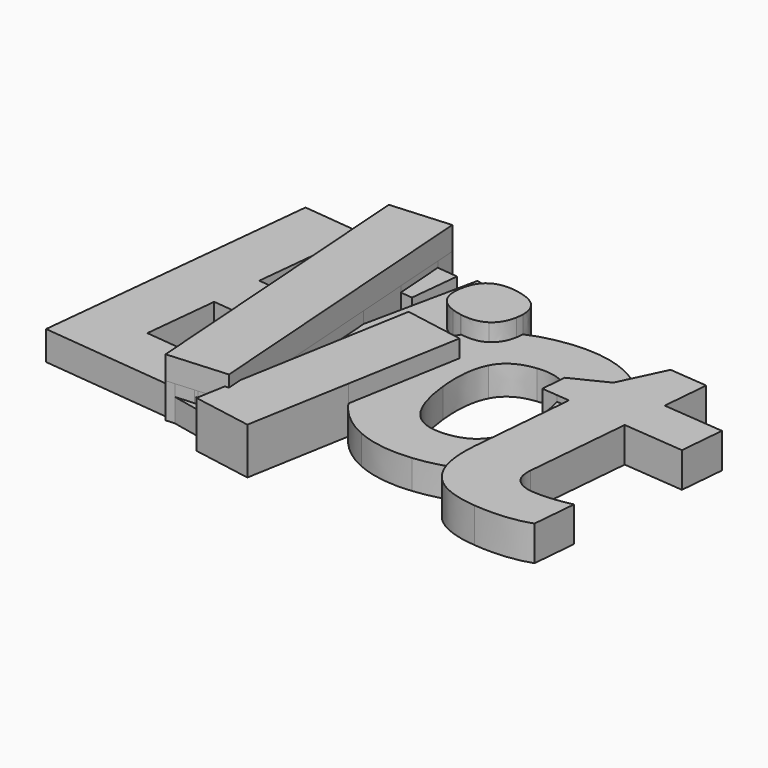
from build123d import *

# Parameters (mm, degrees)
F1_DEPTH = 2.5
F2_DEPTH = 3
F3_DEPTH = 2
F4_DEPTH = 4
F5_DEPTH = 2.5
F6_DEPTH = 3


# Not quite as in the source:
# - a feature names something its author has since deleted; it is built from what else it names


with BuildPart() as f1:
    # F0 (on Top) → F1 (new body)
    with BuildSketch(Plane.XY):
        Polygon((-35.3778718855, -10.0628526476), (-35.0793464958, -10.0938324205), (-35.073883926, -10.0411943399), align=None)
        Polygon((-36.9787601383, -10.1769115417), (-35.3778718855, -10.0628526476), (-37.0800270676, -9.8862097799), (-37.134769104, -10.1437508123), align=None)
        Polygon((-37.0800270676, -9.8862097799), (-35.3778718855, -10.0628526476), (-35.073883926, -10.0411943399), (-34.631335756, -5.7767387725), (-36.1725358308, -5.6167991831), align=None)
        Polygon((-37.7560246741, -9.8160574477), (-37.0800270676, -9.8862097799), (-36.1725358308, -5.6167991831), (-38.0692340227, -5.4199674186), align=None)
        Polygon((-49.2771882306, -8.6204371001), (-37.7560246741, -9.8160574477), (-38.0692340227, -5.4199674186), (-43.6000978097, -4.8459964607), (-42.9404019954, 1.5109239359), (-38.5304347886, 1.0532751491), (-38.8412950671, 5.4163945029), (-42.4957513362, 5.7956393816), (-41.9340578712, 11.2081955427), (-39.2339812879, 10.9279923768), (-39.5448415664, 15.2911117306), (-46.7184868931, 16.0355639968), align=None)
        Polygon((-34.3542809792, 2.9374173386), (-34.8362549846, 0.6699079207), (-34.5922221536, 0.6445831679), align=None)
        Polygon((-38.5304347886, 1.0532751491), (-34.8362549846, 0.6699079207), (-34.3542809792, 2.9374173386), (-34.1475714944, 4.9292986135), (-38.8412950671, 5.4163945029), align=None)
        Polygon((-34.3227687381, 14.7491858653), (-34.0119084596, 10.3860665115), (-32.9652958176, 10.2774532308), (-32.5206451583, 14.5621686765), align=None)
        Polygon((-39.2339812879, 10.9279923768), (-34.0119084596, 10.3860665115), (-34.3227687381, 14.7491858653), (-39.5448415664, 15.2911117306), align=None)
    extrude(amount=F1_DEPTH)

    # F0 (on Top) → F2 (join)
    with BuildSketch(Plane.XY):
        Polygon((-36.9787601383, -10.1769115417), (-35.3778718855, -10.0628526476), (-37.0800270676, -9.8862097799), (-37.134769104, -10.1437508123), align=None)
        Polygon((-37.0800270676, -9.8862097799), (-35.3778718855, -10.0628526476), (-35.073883926, -10.0411943399), (-34.631335756, -5.7767387725), (-36.1725358308, -5.6167991831), align=None)
        Polygon((-34.631335756, -5.7767387725), (-35.073883926, -10.0411943399), (-32.905769146, -9.8867221126), (-32.6648674417, -8.5205006567), (-33.7003912462, 6.0137266645), (-34.3542809792, 2.9374173386), (-34.5922221536, 0.6445831679), (-34.8362549846, 0.6699079207), (-36.1725358308, -5.6167991831), align=None)
        Polygon((-37.134769104, -10.1437508123), (-37.0800270676, -9.8862097799), (-37.7560246741, -9.8160574477), (-37.7265190579, -10.2301873123), (-36.9787601383, -10.1769115417), align=None)
        Polygon((-37.7560246741, -9.8160574477), (-37.0800270676, -9.8862097799), (-36.1725358308, -5.6167991831), (-38.0692340227, -5.4199674186), align=None)
        Polygon((-32.6648674417, -8.5205006567), (-32.905769146, -9.8867221126), (-32.5692362117, -9.8627450647), align=None)
        Polygon((-38.0692340227, -5.4199674186), (-36.1725358308, -5.6167991831), (-34.8362549846, 0.6699079207), (-38.5304347886, 1.0532751491), align=None)
        Polygon((-34.3542809792, 2.9374173386), (-34.8362549846, 0.6699079207), (-34.5922221536, 0.6445831679), align=None)
        Polygon((-38.5304347886, 1.0532751491), (-34.8362549846, 0.6699079207), (-34.3542809792, 2.9374173386), (-34.1475714944, 4.9292986135), (-38.8412950671, 5.4163945029), align=None)
        Polygon((-34.3542809792, 2.9374173386), (-33.7003912462, 6.0137266645), (-34.0119084596, 10.3860665115), (-39.2339812879, 10.9279923768), (-38.8412950671, 5.4163945029), (-34.1475714944, 4.9292986135), align=None)
        Polygon((-39.2339812879, 10.9279923768), (-34.0119084596, 10.3860665115), (-34.3227687381, 14.7491858653), (-39.5448415664, 15.2911117306), align=None)
        Polygon((-39.6015155428, 16.0865666029), (-39.5448415664, 15.2911117306), (-34.3227687381, 14.7491858653), (-34.4442326965, 16.4540088505), align=None)
    extrude(amount=F2_DEPTH)

    # F0 (on Top) + F2_face (on face) → F3 (join)
    with BuildSketch(Plane.XY):
        with BuildLine():
            Line((-33.7003912462, 6.0137266645), (-32.6648674417, -8.5205006567))
            Line((-32.6648674417, -8.5205006567), (-30.0548580187, 6.2815983328))
            Line((-30.0548580187, 6.2815983328), (-28.4189033292, 5.9931353818))
            Line((-28.4189033292, 5.9931353818), (-27.9148304101, 8.3646120143))
            add(Edge.make_bspline(
                [(-27.9148304101, 8.3646120143), (-29.7926134456, 9.0498377198), (-29.4232001055, 11.1448848793)],
                knots=[0.163931303, 0.163931303, 0.163931303, 1, 1, 1], degree=2))
            add(Edge.make_bspline(
                [(-29.4232001055, 11.1448848793), (-29.0403306221, 13.3162456202), (-26.882343227, 13.2220823034)],
                knots=[0, 0, 0, 0.8721015682, 0.8721015682, 0.8721015682], degree=2))
            Line((-26.882343227, 13.2220823034), (-26.5919673681, 14.5881933121))
            Line((-26.5919673681, 14.5881933121), (-31.6493385894, 15.66317075))
            Line((-31.6493385894, 15.66317075), (-33.7003912462, 6.0137266645))
        make_face()
        Polygon((-32.5692362117, -9.8627450647), (-32.905769146, -9.8867221126), (-33.1022277016, -11.0008939476), (-32.0773978827, -11.2187282502), (-28.4189033292, 5.9931353818), (-30.0548580187, 6.2815983328), (-32.6648674417, -8.5205006567), align=None)
        with BuildLine():
            add(Edge.make_bspline(
                [(-27.9148304101, 8.3646120143), (-29.7926134456, 9.0498377198), (-29.4232001055, 11.1448848793)],
                knots=[0.163931303, 0.163931303, 0.163931303, 1, 1, 1], degree=2))
            Line((-27.9148304101, 8.3646120143), (-26.882343227, 13.2220823034))
            add(Edge.make_bspline(
                [(-29.4232001055, 11.1448848793), (-29.0403306221, 13.3162456202), (-26.882343227, 13.2220823034)],
                knots=[0, 0, 0, 0.8721015682, 0.8721015682, 0.8721015682], degree=2))
        make_face()
        Polygon((-35.073883926, -10.0411943399), (-35.0793464958, -10.0938324205), (-35.3778718855, -10.0628526476), (-36.9787601383, -10.1769115417), (-33.1022277016, -11.0008939476), (-32.905769146, -9.8867221126), align=None)
        Polygon((-34.631335756, -5.7767387725), (-35.073883926, -10.0411943399), (-32.905769146, -9.8867221126), (-32.6648674417, -8.5205006567), (-33.7003912462, 6.0137266645), (-34.3542809792, 2.9374173386), (-34.5922221536, 0.6445831679), (-34.8362549846, 0.6699079207), (-36.1725358308, -5.6167991831), align=None)
        Polygon((-34.3542809792, 2.9374173386), (-34.8362549846, 0.6699079207), (-34.5922221536, 0.6445831679), align=None)
    with BuildSketch(Plane(origin=(-36.0853758772, 3.1119107691, 3), x_dir=(1, 0, 0), z_dir=(0, 0, 1))):
        Polygon((-1.6411431807, -13.3420980814), (3.5161396656, -12.9746558338), (1.6411431807, 13.3420980814), (-3.5161396656, 12.9746558338), align=None)
    extrude(amount=F3_DEPTH)

    # F0 (on Top) → F4 (join)
    with BuildSketch(Plane.XY):
        with BuildLine():
            Line((-32.0773978827, -11.2187282502), (-33.1022277016, -11.0008939476))
            Line((-33.1022277016, -11.0008939476), (-33.346561213, -12.3865781485))
            Line((-33.346561213, -12.3865781485), (-28.2547546341, -13.2844010289))
            Line((-28.2547546341, -13.2844010289), (-26.6872976436, -4.3949106953))
            add(Edge.make_bspline(
                [(-26.6872976436, -4.3949106953), (-26.7718769913, -4.2714125894), (-26.8533257577, -4.1437469442)],
                knots=[0.9394626122, 0.9394626122, 0.9394626122, 1, 1, 1], degree=2))
            add(Edge.make_bspline(
                [(-26.8533257577, -4.1437469442), (-28.198754911, -2.0348742315), (-28.5106616753, 0.9327203999)],
                knots=[0, 0, 0, 1, 1, 1], degree=2))
            add(Edge.make_bspline(
                [(-28.5106616753, 0.9327203999), (-28.8097055982, 3.7779332702), (-28.1125120543, 5.9391103334)],
                knots=[0, 0, 0, 0.6160260997, 0.6160260997, 0.6160260997], degree=2))
            Line((-28.1125120543, 5.9391103334), (-28.4189033292, 5.9931353818))
            Line((-28.4189033292, 5.9931353818), (-32.0773978827, -11.2187282502))
        make_face()
        with BuildLine():
            Line((-26.882343227, 13.2220823034), (-27.9148304101, 8.3646120143))
            add(Edge.make_bspline(
                [(-27.0920682235, 8.1501027592), (-27.5466460481, 8.2302570945), (-27.9148304101, 8.3646120143)],
                knots=[0, 0, 0, 0.163931303, 0.163931303, 0.163931303], degree=2))
            add(Edge.make_bspline(
                [(-27.023901472, 8.1384969442), (-27.0578081855, 8.1440617902), (-27.0920682235, 8.1501027592)],
                knots=[0.975337591, 0.975337591, 0.975337591, 1, 1, 1], degree=2))
            add(Edge.make_bspline(
                [(-27.023901472, 8.1384969442), (-26.9422305742, 8.2544564791), (-26.8563287669, 8.3675109901)],
                knots=[0.9598547149, 0.9598547149, 0.9598547149, 1, 1, 1], degree=2))
            add(Edge.make_bspline(
                [(-26.8563287669, 8.3675109901), (-25.6762464221, 9.9206055833), (-23.8176994255, 10.7568832127)],
                knots=[0, 0, 0, 0.5514987826, 0.5514987826, 0.5514987826], degree=2))
            add(Edge.make_bspline(
                [(-26.211203173, 13.145736706), (-23.7840508918, 12.7177642725), (-23.8176994255, 10.7568832127)],
                knots=[0, 0, 0, 0.8752873865, 0.8752873865, 0.8752873865], degree=2))
            add(Edge.make_bspline(
                [(-26.882343227, 13.2220823034), (-26.5658626543, 13.2082727415), (-26.211203173, 13.145736706)],
                knots=[0.8721015682, 0.8721015682, 0.8721015682, 1, 1, 1], degree=2))
        make_face()
        with BuildLine():
            add(Edge.make_bspline(
                [(-27.023901472, 8.1384969442), (-26.9422305742, 8.2544564791), (-26.8563287669, 8.3675109901)],
                knots=[0.9598547149, 0.9598547149, 0.9598547149, 1, 1, 1], degree=2))
            add(Edge.make_bspline(
                [(-24.8946497679, 8.4430052782), (-25.682974387, 7.9184209789), (-27.023901472, 8.1384969442)],
                knots=[0, 0, 0, 0.975337591, 0.975337591, 0.975337591], degree=2))
            add(Edge.make_bspline(
                [(-23.877244986, 10.166983358), (-24.0863915542, 8.9808542283), (-24.8946497679, 8.4430052782)],
                knots=[0, 0, 0, 1, 1, 1], degree=2))
            add(Edge.make_bspline(
                [(-23.8176994255, 10.7568832127), (-23.8224937327, 10.4774931456), (-23.877244986, 10.166983358)],
                knots=[0.8752873865, 0.8752873865, 0.8752873865, 1, 1, 1], degree=2))
            add(Edge.make_bspline(
                [(-26.8563287669, 8.3675109901), (-25.6762464221, 9.9206055833), (-23.8176994255, 10.7568832127)],
                knots=[0, 0, 0, 0.5514987826, 0.5514987826, 0.5514987826], degree=2))
        make_face()
        with BuildLine():
            add(Edge.make_bspline(
                [(-27.9148304101, 8.3646120143), (-29.7926134456, 9.0498377198), (-29.4232001055, 11.1448848793)],
                knots=[0.163931303, 0.163931303, 0.163931303, 1, 1, 1], degree=2))
            Line((-27.9148304101, 8.3646120143), (-26.882343227, 13.2220823034))
            add(Edge.make_bspline(
                [(-29.4232001055, 11.1448848793), (-29.0403306221, 13.3162456202), (-26.882343227, 13.2220823034)],
                knots=[0, 0, 0, 0.8721015682, 0.8721015682, 0.8721015682], degree=2))
        make_face()
        Polygon((-32.5692362117, -9.8627450647), (-32.905769146, -9.8867221126), (-33.1022277016, -11.0008939476), (-32.0773978827, -11.2187282502), (-28.4189033292, 5.9931353818), (-30.0548580187, 6.2815983328), (-32.6648674417, -8.5205006567), align=None)
        with BuildLine():
            add(Edge.make_bspline(
                [(-26.6872976436, -4.3949106953), (-26.7718769913, -4.2714125894), (-26.8533257577, -4.1437469442)],
                knots=[0.9394626122, 0.9394626122, 0.9394626122, 1, 1, 1], degree=2))
            Line((-26.6872976436, -4.3949106953), (-24.9630514398, 5.3837754524))
            Line((-24.9630514398, 5.3837754524), (-28.1125120543, 5.9391103334))
            add(Edge.make_bspline(
                [(-28.5106616753, 0.9327203999), (-28.8097055982, 3.7779332702), (-28.1125120543, 5.9391103334)],
                knots=[0, 0, 0, 0.6160260997, 0.6160260997, 0.6160260997], degree=2))
            add(Edge.make_bspline(
                [(-26.8533257577, -4.1437469442), (-28.198754911, -2.0348742315), (-28.5106616753, 0.9327203999)],
                knots=[0, 0, 0, 1, 1, 1], degree=2))
        make_face()
    extrude(amount=F4_DEPTH)

    # F0 (on Top) → F5 (join)
    with BuildSketch(Plane.XY):
        with BuildLine():
            Line((-24.9630514398, 5.3837754524), (-26.6872976436, -4.3949106953))
            add(Edge.make_bspline(
                [(-23.3082319184, -7.2243041393), (-25.3747346502, -6.3114428972), (-26.6872976436, -4.3949106953)],
                knots=[0, 0, 0, 0.9394626122, 0.9394626122, 0.9394626122], degree=2))
            add(Edge.make_bspline(
                [(-18.3945670513, -7.9107357082), (-21.1085672324, -8.1959886218), (-23.3082319184, -7.2243041393)],
                knots=[0, 0, 0, 1, 1, 1], degree=2))
            add(Edge.make_bspline(
                [(-15.526822019, -7.2607332211), (-16.816191427, -7.7448417453), (-18.3945670513, -7.9107357082)],
                knots=[0.635705233, 0.635705233, 0.635705233, 1, 1, 1], degree=2))
            add(Edge.make_bspline(
                [(-15.526822019, -7.2607332211), (-15.7362478933, -6.1155120567), (-15.6086910396, -4.6575305475)],
                knots=[0.5332842969, 0.5332842969, 0.5332842969, 1, 1, 1], degree=2))
            Line((-15.6086910396, -4.6575305475), (-14.8124113587, 4.4439878531))
            Line((-14.8124113587, 4.4439878531), (-15.9225730211, 4.5411144132))
            add(Edge.make_bspline(
                [(-15.4964103102, 2.3005733372), (-15.6304602981, 3.5759737775), (-15.9225730211, 4.5411144132)],
                knots=[0, 0, 0, 0.455446446, 0.455446446, 0.455446446], degree=2))
            add(Edge.make_bspline(
                [(-15.9517368314, -2.0350954081), (-15.2003824357, -0.5159437493), (-15.4964103102, 2.3005733372)],
                knots=[0, 0, 0, 1, 1, 1], degree=2))
            add(Edge.make_bspline(
                [(-18.7642205893, -3.7708804923), (-16.7030912272, -3.5542470669), (-15.9517368314, -2.0350954081)],
                knots=[0, 0, 0, 1, 1, 1], degree=2))
            add(Edge.make_bspline(
                [(-21.9066614421, -2.652800358), (-20.8361412047, -3.9886481241), (-18.7642205893, -3.7708804923)],
                knots=[0, 0, 0, 1, 1, 1], degree=2))
            add(Edge.make_bspline(
                [(-23.2715082443, 1.4833776147), (-22.9771816795, -1.316952592), (-21.9066614421, -2.652800358)],
                knots=[0, 0, 0, 1, 1, 1], degree=2))
            add(Edge.make_bspline(
                [(-22.8019878506, 5.7878068067), (-23.5675361188, 4.2998947012), (-23.2715082443, 1.4833776147)],
                knots=[0, 0, 0, 1, 1, 1], degree=2))
            add(Edge.make_bspline(
                [(-19.9807058469, 7.4917852345), (-22.0364395824, 7.2757189123), (-22.8019878506, 5.7878068067)],
                knots=[0, 0, 0, 1, 1, 1], degree=2))
            add(Edge.make_bspline(
                [(-17.1000146463, 6.6820511263), (-18.139176229, 7.6853377967), (-19.9807058469, 7.4917852345)],
                knots=[0.1135054063, 0.1135054063, 0.1135054063, 1, 1, 1], degree=2))
            Line((-17.1000146463, 6.6820511263), (-17.0863969164, 6.8377024908))
            Line((-17.0863969164, 6.8377024908), (-14.0980890907, 8.3135561352))
            Line((-14.0980890907, 8.3135561352), (-13.4336721304, 9.710496258))
            add(Edge.make_bspline(
                [(-15.433567304, 10.9673584912), (-14.3249420181, 10.4828209599), (-13.4336721304, 9.710496258)],
                knots=[0, 0, 0, 0.5042574102, 0.5042574102, 0.5042574102], degree=2))
            add(Edge.make_bspline(
                [(-20.3460979647, 11.6429988069), (-17.6320977836, 11.9282517204), (-15.433567304, 10.9673584912)],
                knots=[0, 0, 0, 1, 1, 1], degree=2))
            add(Edge.make_bspline(
                [(-23.8176994255, 10.7568832127), (-22.3062534954, 11.4369781588), (-20.3460979647, 11.6429988069)],
                knots=[0.5514987826, 0.5514987826, 0.5514987826, 1, 1, 1], degree=2))
            add(Edge.make_bspline(
                [(-23.8176994255, 10.7568832127), (-23.8224937327, 10.4774931456), (-23.877244986, 10.166983358)],
                knots=[0.8752873865, 0.8752873865, 0.8752873865, 1, 1, 1], degree=2))
            add(Edge.make_bspline(
                [(-23.877244986, 10.166983358), (-24.0863915542, 8.9808542283), (-24.8946497679, 8.4430052782)],
                knots=[0, 0, 0, 1, 1, 1], degree=2))
            add(Edge.make_bspline(
                [(-24.8946497679, 8.4430052782), (-25.682974387, 7.9184209789), (-27.023901472, 8.1384969442)],
                knots=[0, 0, 0, 0.975337591, 0.975337591, 0.975337591], degree=2))
            add(Edge.make_bspline(
                [(-28.1125120543, 5.9391103334), (-27.723380667, 7.1453490259), (-27.023901472, 8.1384969442)],
                knots=[0.6160260997, 0.6160260997, 0.6160260997, 0.9598547149, 0.9598547149, 0.9598547149], degree=2))
            Line((-28.1125120543, 5.9391103334), (-24.9630514398, 5.3837754524))
        make_face()
        with BuildLine():
            add(Edge.make_bspline(
                [(-15.526822019, -7.2607332211), (-15.7362478933, -6.1155120567), (-15.6086910396, -4.6575305475)],
                knots=[0.5332842969, 0.5332842969, 0.5332842969, 1, 1, 1], degree=2))
            add(Edge.make_bspline(
                [(-11.906907113, -4.6021611797), (-13.2768339483, -6.4159494084), (-15.526822019, -7.2607332211)],
                knots=[0, 0, 0, 0.635705233, 0.635705233, 0.635705233], degree=2))
            add(Edge.make_bspline(
                [(-10.2356743727, 2.8534989648), (-9.7519353365, -1.7489705271), (-11.906907113, -4.6021611797)],
                knots=[0, 0, 0, 1, 1, 1], degree=2))
            add(Edge.make_bspline(
                [(-11.8913089808, 7.9137794291), (-10.547581137, 5.8210935962), (-10.2356743727, 2.8534989648)],
                knots=[0, 0, 0, 1, 1, 1], degree=2))
            add(Edge.make_bspline(
                [(-13.4336721304, 9.710496258), (-12.557452102, 8.9512129235), (-11.8913089808, 7.9137794291)],
                knots=[0.5042574102, 0.5042574102, 0.5042574102, 1, 1, 1], degree=2))
            Line((-13.4336721304, 9.710496258), (-14.0980890907, 8.3135561352))
            Line((-14.0980890907, 8.3135561352), (-17.0863969164, 6.8377024908))
            Line((-17.0863969164, 6.8377024908), (-17.1000146463, 6.6820511263))
            add(Edge.make_bspline(
                [(-16.84706324, 6.4055117567), (-16.9669619932, 6.5535918419), (-17.1000146463, 6.6820511263)],
                knots=[0, 0, 0, 0.1135054063, 0.1135054063, 0.1135054063], degree=2))
            add(Edge.make_bspline(
                [(-15.9225730211, 4.5411144132), (-16.2718369638, 5.6950827178), (-16.84706324, 6.4055117567)],
                knots=[0.455446446, 0.455446446, 0.455446446, 1, 1, 1], degree=2))
            Line((-15.9225730211, 4.5411144132), (-14.8124113587, 4.4439878531))
            Line((-14.8124113587, 4.4439878531), (-15.6086910396, -4.6575305475))
        make_face()
        with BuildLine():
            add(Edge.make_bspline(
                [(-26.6872976436, -4.3949106953), (-26.7718769913, -4.2714125894), (-26.8533257577, -4.1437469442)],
                knots=[0.9394626122, 0.9394626122, 0.9394626122, 1, 1, 1], degree=2))
            Line((-26.6872976436, -4.3949106953), (-24.9630514398, 5.3837754524))
            Line((-24.9630514398, 5.3837754524), (-28.1125120543, 5.9391103334))
            add(Edge.make_bspline(
                [(-28.5106616753, 0.9327203999), (-28.8097055982, 3.7779332702), (-28.1125120543, 5.9391103334)],
                knots=[0, 0, 0, 0.6160260997, 0.6160260997, 0.6160260997], degree=2))
            add(Edge.make_bspline(
                [(-26.8533257577, -4.1437469442), (-28.198754911, -2.0348742315), (-28.5106616753, 0.9327203999)],
                knots=[0, 0, 0, 1, 1, 1], degree=2))
        make_face()
        with BuildLine():
            add(Edge.make_bspline(
                [(-27.023901472, 8.1384969442), (-26.9422305742, 8.2544564791), (-26.8563287669, 8.3675109901)],
                knots=[0.9598547149, 0.9598547149, 0.9598547149, 1, 1, 1], degree=2))
            add(Edge.make_bspline(
                [(-24.8946497679, 8.4430052782), (-25.682974387, 7.9184209789), (-27.023901472, 8.1384969442)],
                knots=[0, 0, 0, 0.975337591, 0.975337591, 0.975337591], degree=2))
            add(Edge.make_bspline(
                [(-23.877244986, 10.166983358), (-24.0863915542, 8.9808542283), (-24.8946497679, 8.4430052782)],
                knots=[0, 0, 0, 1, 1, 1], degree=2))
            add(Edge.make_bspline(
                [(-23.8176994255, 10.7568832127), (-23.8224937327, 10.4774931456), (-23.877244986, 10.166983358)],
                knots=[0.8752873865, 0.8752873865, 0.8752873865, 1, 1, 1], degree=2))
            add(Edge.make_bspline(
                [(-26.8563287669, 8.3675109901), (-25.6762464221, 9.9206055833), (-23.8176994255, 10.7568832127)],
                knots=[0, 0, 0, 0.5514987826, 0.5514987826, 0.5514987826], degree=2))
        make_face()
    extrude(amount=F5_DEPTH)

    # F0 (on Top) → F6 (join)
    with BuildSketch(Plane.XY):
        with BuildLine():
            add(Edge.make_bspline(
                [(-11.906907113, -4.6021611797), (-13.2768339483, -6.4159494084), (-15.526822019, -7.2607332211)],
                knots=[0, 0, 0, 0.635705233, 0.635705233, 0.635705233], degree=2))
            add(Edge.make_bspline(
                [(-14.6082613013, -9.4695235458), (-15.2875253136, -8.5692995697), (-15.526822019, -7.2607332211)],
                knots=[0, 0, 0, 0.5332842969, 0.5332842969, 0.5332842969], degree=2))
            add(Edge.make_bspline(
                [(-10.2430345436, -11.4280690037), (-13.3345241665, -11.1575987083), (-14.6082613013, -9.4695235458)],
                knots=[0, 0, 0, 1, 1, 1], degree=2))
            add(Edge.make_bspline(
                [(-5.438264146, -10.9770605576), (-7.4379941339, -11.6734782403), (-10.2430345436, -11.4280690037)],
                knots=[0, 0, 0, 1, 1, 1], degree=2))
            Line((-5.438264146, -10.9770605576), (-5.1030133778, -7.1451267417))
            add(Edge.make_bspline(
                [(-8.3973753288, -7.4505291747), (-7.0461997943, -7.5687417164), (-5.1030133778, -7.1451267417)],
                knots=[0, 0, 0, 1, 1, 1], degree=2))
            add(Edge.make_bspline(
                [(-9.9837289083, -6.7834723169), (-9.4134593308, -7.3616333433), (-8.3973753288, -7.4505291747)],
                knots=[0, 0, 0, 1, 1, 1], degree=2))
            add(Edge.make_bspline(
                [(-10.458009902, -5.1081567565), (-10.5539984859, -6.2053112905), (-9.9837289083, -6.7834723169)],
                knots=[0, 0, 0, 1, 1, 1], degree=2))
            Line((-10.458009902, -5.1081567565), (-9.6617302211, 3.9933616441))
            Line((-9.6617302211, 3.9933616441), (-4.3759315301, 3.5309141809))
            Line((-4.3759315301, 3.5309141809), (-4.0373708106, 7.4006809118))
            Line((-4.0373708106, 7.4006809118), (-9.3231695017, 7.8631283749))
            Line((-9.3231695017, 7.8631283749), (-8.9713689776, 11.8842267657))
            Line((-8.9713689776, 11.8842267657), (-12.2628325796, 12.1721925173))
            Line((-12.2628325796, 12.1721925173), (-13.4336721304, 9.710496258))
            add(Edge.make_bspline(
                [(-13.4336721304, 9.710496258), (-12.557452102, 8.9512129235), (-11.8913089808, 7.9137794291)],
                knots=[0.5042574102, 0.5042574102, 0.5042574102, 1, 1, 1], degree=2))
            add(Edge.make_bspline(
                [(-11.8913089808, 7.9137794291), (-10.547581137, 5.8210935962), (-10.2356743727, 2.8534989648)],
                knots=[0, 0, 0, 1, 1, 1], degree=2))
            add(Edge.make_bspline(
                [(-10.2356743727, 2.8534989648), (-9.7519353365, -1.7489705271), (-11.906907113, -4.6021611797)],
                knots=[0, 0, 0, 1, 1, 1], degree=2))
        make_face()
        with BuildLine():
            add(Edge.make_bspline(
                [(-15.526822019, -7.2607332211), (-15.7362478933, -6.1155120567), (-15.6086910396, -4.6575305475)],
                knots=[0.5332842969, 0.5332842969, 0.5332842969, 1, 1, 1], degree=2))
            add(Edge.make_bspline(
                [(-11.906907113, -4.6021611797), (-13.2768339483, -6.4159494084), (-15.526822019, -7.2607332211)],
                knots=[0, 0, 0, 0.635705233, 0.635705233, 0.635705233], degree=2))
            add(Edge.make_bspline(
                [(-10.2356743727, 2.8534989648), (-9.7519353365, -1.7489705271), (-11.906907113, -4.6021611797)],
                knots=[0, 0, 0, 1, 1, 1], degree=2))
            add(Edge.make_bspline(
                [(-11.8913089808, 7.9137794291), (-10.547581137, 5.8210935962), (-10.2356743727, 2.8534989648)],
                knots=[0, 0, 0, 1, 1, 1], degree=2))
            add(Edge.make_bspline(
                [(-13.4336721304, 9.710496258), (-12.557452102, 8.9512129235), (-11.8913089808, 7.9137794291)],
                knots=[0.5042574102, 0.5042574102, 0.5042574102, 1, 1, 1], degree=2))
            Line((-13.4336721304, 9.710496258), (-14.0980890907, 8.3135561352))
            Line((-14.0980890907, 8.3135561352), (-17.0863969164, 6.8377024908))
            Line((-17.0863969164, 6.8377024908), (-17.1000146463, 6.6820511263))
            add(Edge.make_bspline(
                [(-16.84706324, 6.4055117567), (-16.9669619932, 6.5535918419), (-17.1000146463, 6.6820511263)],
                knots=[0, 0, 0, 0.1135054063, 0.1135054063, 0.1135054063], degree=2))
            add(Edge.make_bspline(
                [(-15.9225730211, 4.5411144132), (-16.2718369638, 5.6950827178), (-16.84706324, 6.4055117567)],
                knots=[0.455446446, 0.455446446, 0.455446446, 1, 1, 1], degree=2))
            Line((-15.9225730211, 4.5411144132), (-14.8124113587, 4.4439878531))
            Line((-14.8124113587, 4.4439878531), (-15.6086910396, -4.6575305475))
        make_face()
        with BuildLine():
            Line((-17.2769555337, 4.6596075291), (-15.9225730211, 4.5411144132))
            add(Edge.make_bspline(
                [(-15.9225730211, 4.5411144132), (-16.2718369638, 5.6950827178), (-16.84706324, 6.4055117567)],
                knots=[0.455446446, 0.455446446, 0.455446446, 1, 1, 1], degree=2))
            add(Edge.make_bspline(
                [(-16.84706324, 6.4055117567), (-16.9669619932, 6.5535918419), (-17.1000146463, 6.6820511263)],
                knots=[0, 0, 0, 0.1135054063, 0.1135054063, 0.1135054063], degree=2))
            Line((-17.1000146463, 6.6820511263), (-17.2769555337, 4.6596075291))
        make_face()
    extrude(amount=F6_DEPTH)


solid = f1.part
